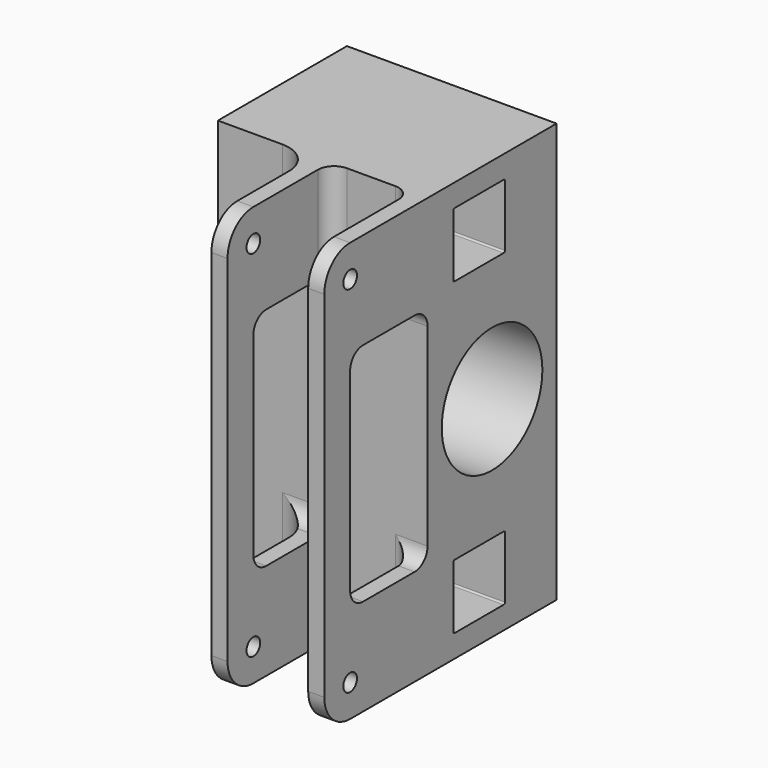
from build123d import *

# Parameters (mm, degrees)
F1_DEPTH = 130
F2_R     = 2.65
F2_R_2   = 13
F2_R_3   = 1.75
F3_DEPTH = 80
F2_R_4   = 19.5
F4_DEPTH = 53
F5_R     = 10
F6_R     = 5
F7_SIZE  = 2
F8_R     = 2
F9_DEPTH = 15


# Not quite as in the source:
# - a feature names something its author has since deleted; it is built from what else it names


with BuildPart() as f1:
    # F0 (on Top) → F1 (new body)
    with BuildSketch(Plane.XY):
        Polygon((35, 90), (-30, 90), (-30, 40), (0, 40), (0, 0), (5, 0), (5, 40), (30, 40), (30, 0), (35, 0), align=None)
    extrude(amount=F1_DEPTH)

    # F2 (on face) → F3 (cut)
    with BuildSketch(Plane.YZ.offset(35)):
        with Locations((10, 120)):
            Circle(F2_R)
        with Locations((10, 10)):
            Circle(F2_R)
        with BuildLine():
            ThreePointArc((10, 35), (11.4644660941, 31.4644660941), (15, 30))
            Line((15, 30), (35, 30))
            ThreePointArc((35, 30), (38.5355339059, 31.4644660941), (40, 35))
            Line((40, 35), (40, 95))
            ThreePointArc((40, 95), (38.5355339059, 98.5355339059), (35, 100))
            Line((35, 100), (15, 100))
            ThreePointArc((15, 100), (11.4644660941, 98.5355339059), (10, 95))
            Line((10, 95), (10, 35))
        make_face()
        with Locations((65, 65)):
            Circle(F2_R_2)
        with Locations((65, 49.5)):
            Circle(F2_R_3)
        with Locations((51.5766062413, 57.25)):
            Circle(F2_R_3)
        with Locations((51.5766062413, 72.75)):
            Circle(F2_R_3)
        with Locations((65, 80.5)):
            Circle(F2_R_3)
        with Locations((78.4233937587, 72.75)):
            Circle(F2_R_3)
        with Locations((78.4233937587, 57.25)):
            Circle(F2_R_3)
        with BuildLine():
            Line((50, 26.5), (50, 7.5))
            ThreePointArc((50, 7.5), (50.1464466094, 7.1464466094), (50.5, 7))
            Line((50.5, 7), (69.5, 7))
            ThreePointArc((69.5, 7), (69.8535533906, 7.1464466094), (70, 7.5))
            Line((70, 7.5), (70, 26.5))
            ThreePointArc((70, 26.5), (69.8535533906, 26.8535533906), (69.5, 27))
            Line((69.5, 27), (50.5, 27))
            ThreePointArc((50.5, 27), (50.1464466094, 26.8535533906), (50, 26.5))
        make_face()
        with BuildLine():
            ThreePointArc((50, 103.5), (50.1464466094, 103.1464466094), (50.5, 103))
            Line((50.5, 103), (69.5, 103))
            ThreePointArc((69.5, 103), (69.8535533906, 103.1464466094), (70, 103.5))
            Line((70, 103.5), (70, 122.5))
            ThreePointArc((70, 122.5), (69.8535533906, 122.8535533906), (69.5, 123))
            Line((69.5, 123), (50.5, 123))
            ThreePointArc((50.5, 123), (50.1464466094, 122.8535533906), (50, 122.5))
            Line((50, 122.5), (50, 103.5))
        make_face()
    extrude(amount=-F3_DEPTH, mode=Mode.SUBTRACT)

    # F2 (on face) → F4 (cut)
    with BuildSketch(Plane.YZ.offset(35)):
        with Locations((65, 65)):
            Circle(F2_R_4)
        with Locations((51.5766062413, 57.25)):
            Circle(F2_R_3, mode=Mode.SUBTRACT)
        with Locations((65, 49.5)):
            Circle(F2_R_3, mode=Mode.SUBTRACT)
        with Locations((78.4233937587, 57.25)):
            Circle(F2_R_3, mode=Mode.SUBTRACT)
        with Locations((51.5766062413, 72.75)):
            Circle(F2_R_3, mode=Mode.SUBTRACT)
        with Locations((65, 65)):
            Circle(F2_R_2, mode=Mode.SUBTRACT)
        with Locations((65, 80.5)):
            Circle(F2_R_3, mode=Mode.SUBTRACT)
        with Locations((78.4233937587, 72.75)):
            Circle(F2_R_3, mode=Mode.SUBTRACT)
    extrude(amount=-F4_DEPTH, mode=Mode.SUBTRACT)

    # F5
    f5_edges = [f1.edges().sort_by_distance(p)[0] for p in [
        (32.5, 0, 130),
        (2.5, 0, 130),
        (32.5, 0, 0),
        (2.5, 0, 0),
        (0, 40, 112.5),
        (0, 40, 17.5),
    ]]
    fillet(f5_edges, radius=F5_R)

    # F6
    f6_edges = [f1.edges().sort_by_distance(p)[0] for p in [
        (5, 40, 112.5),
        (5, 40, 17.5),
        (30, 40, 112.5),
        (30, 40, 17.5),
    ]]
    fillet(f6_edges, radius=F6_R)

    # F7
    f7_edges = [f1.edges().sort_by_distance(p)[0] for p in [
        (-30, 60, 123),
        (-30, 60, 27),
    ]]
    chamfer(f7_edges, length=F7_SIZE)

    # F8 (on face) → F9 (cut)
    with BuildSketch(Plane(origin=(0, 90, 0), x_dir=(-1, 0, 0), z_dir=(0, 1, 0))):
        with Locations((21, 10)):
            Circle(F8_R)
        with Locations((1, 10)):
            Circle(F8_R)
        with Locations((-19, 10)):
            Circle(F8_R)
        with Locations((1, 35)):
            Circle(F8_R)
        with Locations((-19, 35)):
            Circle(F8_R)
        with Locations((21, 35)):
            Circle(F8_R)
        with Locations((21, 95)):
            Circle(F8_R)
        with Locations((1, 95)):
            Circle(F8_R)
        with Locations((-19, 95)):
            Circle(F8_R)
        with Locations((-19, 120)):
            Circle(F8_R)
        with Locations((1, 120)):
            Circle(F8_R)
        with Locations((21, 120)):
            Circle(F8_R)
    extrude(amount=-F9_DEPTH, mode=Mode.SUBTRACT)


solid = f1.part
